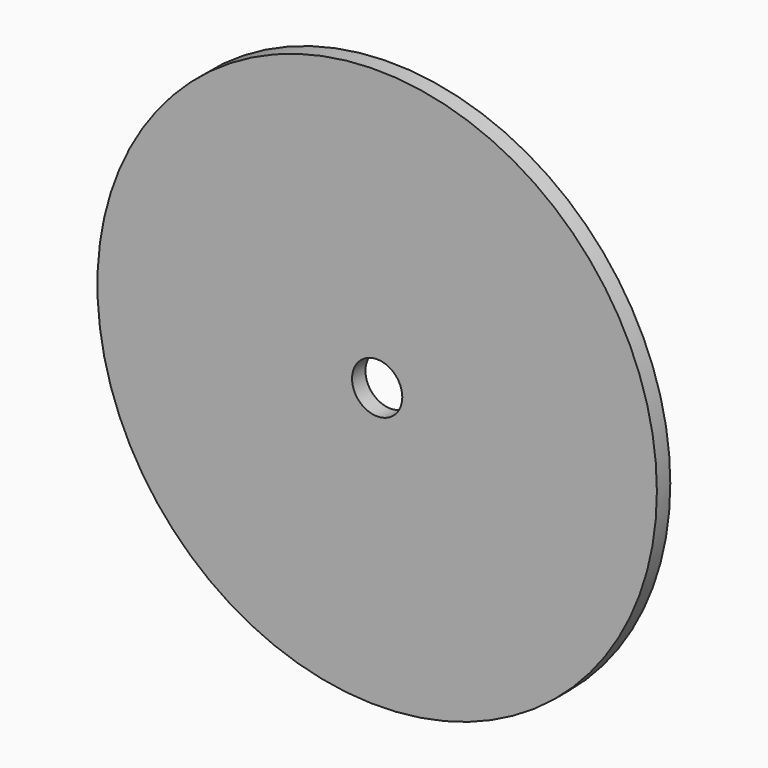
from build123d import *

# Parameters (mm, degrees)
F0_R     = 50.1
F0_R_2   = 4.5
F2_DEPTH = 3


# Not quite as in the source:
# - the program builds the solid bodies; features that only make, move or delete a surface that nothing else refers to are left out


with BuildPart() as f2:
    # F0 (on Front) → F2 (new body)
    with BuildSketch(Plane.XZ):
        Circle(F0_R)
        Circle(F0_R_2, mode=Mode.SUBTRACT)
    extrude(amount=F2_DEPTH)


solid = f2.part
